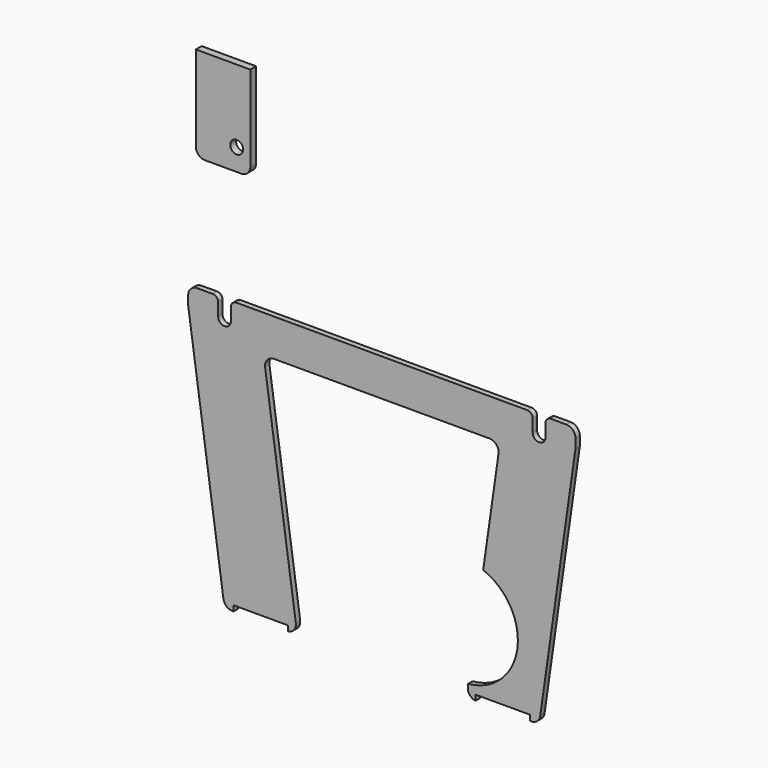
from build123d import *

# Parameters (mm, degrees)
F1_DEPTH     = 3
F2_W         = 30
F2_H         = 3
F3_DEPTH     = 25
F4_W         = 30
F4_H         = 52
F5_DEPTH     = 4
F6_D         = 7.1
F7_T1_DEPTH  = 3
F7_T3_DEPTH  = 3
F7_T5_DEPTH  = 28
F7_T7_DEPTH  = 28
F7_T9_DEPTH  = 24.6823850424
F7_T11_DEPTH = 31.5342712156
F7_T13_DEPTH = 31.5342712156
F7_T15_DEPTH = 24.6823850424
F8_R         = 3
F9_R         = 5


# Not quite as in the source:
# - a fillet or chamfer that OpenCascade refuses, or shapes differently, is made with other operations: its cross-section is extruded or revolved along the edge and cut away or added


with BuildPart() as f1:
    # F0 (on Front) → F1 (new body)
    with BuildSketch(Plane.XZ):
        with BuildLine():
            Line((-20, 10), (-20, 0))
            Line((-20, 0), (0, -140))
            Line((0, -140), (40, -140))
            Line((40, -140), (21.5, -10.5))
            Line((21.5, -10.5), (151.5, -10.5))
            Line((151.5, -10.5), (142.25, -75.25))
            ThreePointArc((142.25, -75.25), (161.0212778612, -107.4317915028), (133.9899494937, -133.0703535444))
            Line((133.9899494937, -133.0703535444), (133, -140))
            Line((133, -140), (173, -140))
            Line((173, -140), (193, 0))
            Line((193, 0), (193, 10))
            Line((193, 10), (176.5, 10))
            Line((176.5, 10), (176.5, 0))
            ThreePointArc((176.5, 0), (173, -3.5), (169.5, 0))
            Line((169.5, 0), (169.5, 10))
            Line((169.5, 10), (153, 10))
            Line((153, 10), (20, 10))
            Line((20, 10), (3.5, 10))
            Line((3.5, 10), (3.5, 0))
            ThreePointArc((3.5, 0), (0, -3.5), (-3.5, 0))
            Line((-3.5, 0), (-3.5, 10))
            Line((-3.5, 10), (-20, 10))
        make_face()
    extrude(amount=F1_DEPTH)

    # F2 (on face) → F3 (cut)
    with BuildSketch(Plane.XZ.offset(3)):
        with Locations((20, -138.5)):
            Rectangle(F2_W, F2_H)
        with Locations((153, -138.5)):
            Rectangle(F2_W, F2_H)
    extrude(amount=-F3_DEPTH, mode=Mode.SUBTRACT)

    # F7: fillet of radius 5 on 8 edges, made by hand

    # F7_s2 → F7_t1 (join)
    with BuildSketch(Plane.XZ):
        with BuildLine():
            ThreePointArc((150.6846990313, -16.2071067812), (149.5122213379, -12.2239912932), (145.734951563, -10.5))
            Line((145.734951563, -10.5), (151.5, -10.5))
            Line((151.5, -10.5), (150.6846990313, -16.2071067812))
        make_face()
    extrude(amount=F7_T1_DEPTH)

    # F7_s4 → F7_t3 (join)
    with BuildSketch(Plane.XZ):
        with BuildLine():
            ThreePointArc((27.265048437, -10.5), (23.4877786621, -12.2239912932), (22.3153009687, -16.2071067812))
            Line((22.3153009687, -16.2071067812), (21.5, -10.5))
            Line((21.5, -10.5), (27.265048437, -10.5))
        make_face()
    extrude(amount=F7_T3_DEPTH)

    # F7_s6 → F7_t5 (cut)
    with BuildSketch(Plane.XZ.offset(-12.5)):
        with BuildLine():
            ThreePointArc((-15, 10), (-18.5355339059, 8.5355339059), (-20, 5))
            Line((-20, 5), (-20, 10))
            Line((-20, 10), (-15, 10))
        make_face()
    extrude(amount=F7_T5_DEPTH, mode=Mode.SUBTRACT)

    # F7_s8 → F7_t7 (cut)
    with BuildSketch(Plane.XZ.offset(-12.5)):
        with BuildLine():
            ThreePointArc((188, 10), (191.5355339059, 8.5355339059), (193, 5))
            Line((193, 5), (193, 10))
            Line((193, 10), (188, 10))
        make_face()
    extrude(amount=F7_T7_DEPTH, mode=Mode.SUBTRACT)

    # F7_s10 → F7_t9 (cut)
    with BuildSketch(Plane.XZ.offset(-10.8411925212)):
        with BuildLine():
            ThreePointArc((173.6132704598, -135.7071067812), (171.9395316983, -138.777269775), (168.6635229915, -140))
            Line((168.6635229915, -140), (173, -140))
            Line((173, -140), (173.6132704598, -135.7071067812))
        make_face()
    extrude(amount=F7_T9_DEPTH, mode=Mode.SUBTRACT)

    # F7_s12 → F7_t11 (cut)
    with BuildSketch(Plane.XZ.offset(-14.2671356078)):
        with BuildLine():
            ThreePointArc((138, -140), (134.7417930933, -138.0374701654), (133.8070710669, -134.3505025316))
            Line((133.8070710669, -134.3505025316), (133, -140))
            Line((133, -140), (138, -140))
        make_face()
    extrude(amount=F7_T11_DEPTH, mode=Mode.SUBTRACT)

    # F7_s14 → F7_t13 (cut)
    with BuildSketch(Plane.XZ.offset(-14.2671356078)):
        with BuildLine():
            ThreePointArc((39.1929289331, -134.3505025316), (38.2582069067, -138.0374701654), (35, -140))
            Line((35, -140), (40, -140))
            Line((40, -140), (39.1929289331, -134.3505025316))
        make_face()
    extrude(amount=F7_T13_DEPTH, mode=Mode.SUBTRACT)

    # F7_s16 → F7_t15 (cut)
    with BuildSketch(Plane.XZ.offset(-10.8411925212)):
        with BuildLine():
            ThreePointArc((4.3364770085, -140), (1.0604683017, -138.777269775), (-0.6132704598, -135.7071067812))
            Line((-0.6132704598, -135.7071067812), (0, -140))
            Line((0, -140), (4.3364770085, -140))
        make_face()
    extrude(amount=F7_T15_DEPTH, mode=Mode.SUBTRACT)

    # F8
    f8_edges = [f1.edges().sort_by_distance(p)[0] for p in [
        (169.5, -1.5, 10),
        (176.5, -1.5, 10),
        (-3.5, -1.5, 10),
        (3.5, -1.5, 10),
    ]]
    fillet(f8_edges, radius=F8_R)


with BuildPart() as f5:
    # F4 (on Front) → F5 (new body)
    with BuildSketch(Plane.XZ):
        with Locations((0, 100)):
            Rectangle(F4_W, F4_H)
    extrude(amount=F5_DEPTH)

    # F6 (through all)
    with Locations(Plane(origin=(0, 0, 0), x_dir=(1, 0, 0), z_dir=(0, 1, 0))):
        with Locations((7.5, -86)):
            Hole(F6_D / 2)

    # F9
    f9_edges = [f5.edges().sort_by_distance(p)[0] for p in [
        (-15, -2, 74),
        (15, -2, 74),
    ]]
    fillet(f9_edges, radius=F9_R)


solid = Compound([f1.part, f5.part])
